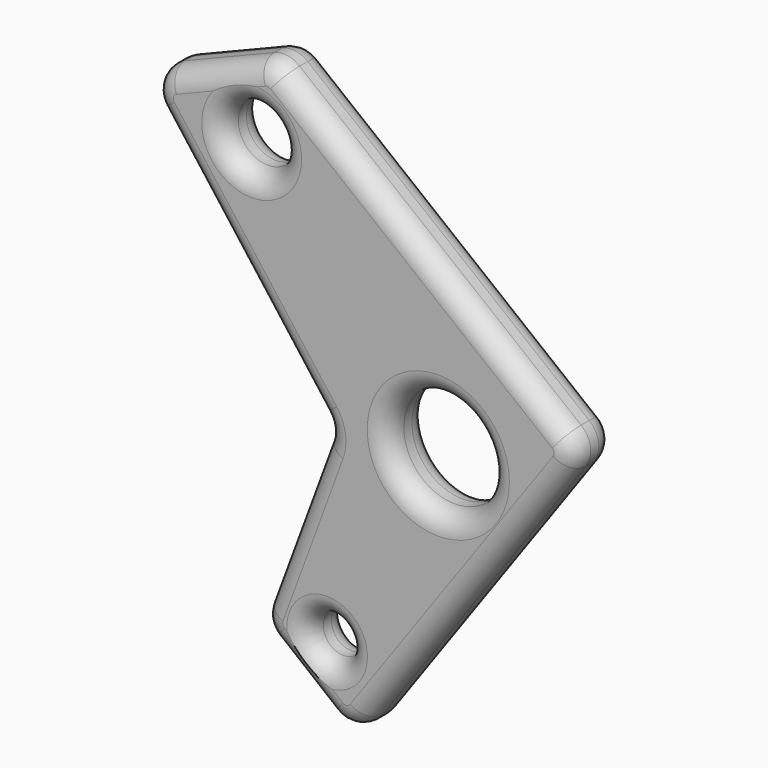
from build123d import *

# Parameters (mm, degrees)
F0_R         = 5.0114511668
F0_R_2       = 12.7
F0_R_3       = 7.4050061566
F1_DEPTH     = 12.7
F2_T1_DEPTH  = 67.4832294606
F2_T3_DEPTH  = 43.3480770651
F2_T5_DEPTH  = 18.6902227842
F2_T7_DEPTH  = 87.4726302362
F2_T9_DEPTH  = 90.1056698852
F2_T11_DEPTH = 24.0510688963
F2_T14_ANGLE = 104.9172533531
F2_T16_ANGLE = 57.3091059371
F2_T18_ANGLE = 71.4094727033
F2_T20_ANGLE = 93.3635037829
F2_T22_ANGLE = 86.9511700386
F2_T24_ANGLE = 60.6677060592
F3_T1_DEPTH  = 67.4832294606
F3_T3_DEPTH  = 43.3480770651
F3_T5_DEPTH  = 18.6902227842
F3_T7_DEPTH  = 87.4726302362
F3_T9_DEPTH  = 90.1056698852
F3_T11_DEPTH = 24.0510688963
F3_T14_ANGLE = 104.9172533531
F3_T16_ANGLE = 57.3091059371
F3_T18_ANGLE = 71.4094727033
F3_T20_ANGLE = 93.3635037829
F3_T22_ANGLE = 86.9511700386
F3_T24_ANGLE = 60.6677060592


# Not quite as in the source:
# - a fillet or chamfer that OpenCascade refuses, or shapes differently, is made with other operations: its cross-section is extruded or revolved along the edge and cut away or added


with BuildPart() as f1:
    # F0 (on Front) → F1 (new body)
    with BuildSketch(Plane.XZ):
        with BuildLine():
            Line((-70.0973556896, 53.2575167822), (-29.4707006051, -0.6262577244))
            ThreePointArc((-29.4707006051, -0.6262577244), (-28.258510501, -3.5258173929), (-28.5852000675, -6.6515373175))
            Line((-28.5852000675, -6.6515373175), (-43.6199162753, -47.3088010447))
            ThreePointArc((-43.6199162753, -47.3088010447), (-43.7857787204, -51.1986473183), (-41.6503181511, -54.4541384548))
            Line((-41.6503181511, -54.4541384548), (-27.101605684, -66.1869724377))
            ThreePointArc((-27.101605684, -66.1869724377), (-22.2538851697, -67.5353399701), (-17.947095407, -64.9334077788))
            Line((-17.947095407, -64.9334077788), (32.8746118318, 6.2607992451))
            ThreePointArc((32.8746118318, 6.2607992451), (33.9952305909, 10.8289222441), (31.6653512614, 14.9148978249))
            Line((31.6653512614, 14.9148978249), (-38.7836697055, 71.0928934304))
            ThreePointArc((-38.7836697055, 71.0928934304), (-41.8330514714, 72.4126619619), (-45.1314974688, 72.0116979572))
            Line((-45.1314974688, 72.0116979572), (-67.4158361597, 62.9639267308))
            ThreePointArc((-67.4158361597, 62.9639267308), (-71.1477537613, 58.7713096023), (-70.0973556896, 53.2575167822))
        make_face()
        with Locations((-27.8284879681, -50.1332112049)):
            Circle(F0_R, mode=Mode.SUBTRACT)
        Circle(F0_R_2, mode=Mode.SUBTRACT)
        with Locations((-46.6999868111, 54.0848947769)):
            Circle(F0_R_3, mode=Mode.SUBTRACT)
    extrude(amount=F1_DEPTH)

    # F2: fillet of radius 5.08 on 15 edges, made by hand

    # F2_s2 → F2_t1 (cut)
    with BuildSketch(Plane(origin=(-51.0068312032, 0, 67.6511660912), x_dir=(0, 1, 0), z_dir=(0.6020259464, 0, -0.7984765243))):
        with BuildLine():
            ThreePointArc((-7.62, -23.9086859864), (-11.2121024484, -22.4207884348), (-12.7, -18.8286859864))
            Line((-12.7, -18.8286859864), (-12.7, -23.9086859864))
            Line((-12.7, -23.9086859864), (-7.62, -23.9086859864))
        make_face()
    extrude(amount=F2_T1_DEPTH, mode=Mode.SUBTRACT)

    # F2_s4 → F2_t3 (cut)
    with BuildSketch(Plane(origin=(-5.6024752773, 0, -15.1503567959), x_dir=(0, 1, 0), z_dir=(-0.3468369816, 0, -0.9379254278))):
        with BuildLine():
            ThreePointArc((-7.62, -24.5037868769), (-11.2121024484, -23.0158893253), (-12.7, -19.4237868769))
            Line((-12.7, -19.4237868769), (-12.7, -24.5037868769))
            Line((-12.7, -24.5037868769), (-7.62, -24.5037868769))
        make_face()
    extrude(amount=F2_T3_DEPTH, mode=Mode.SUBTRACT)

    # F2_s6 → F2_t5 (cut)
    with BuildSketch(Plane(origin=(1.3720089605, 0, -1.1064589662), x_dir=(0, 1, 0), z_dir=(0.7784130042, 0, -0.6277524949))):
        with BuildLine():
            ThreePointArc((-7.62, -68.5339006399), (-11.2121024484, -67.0460030883), (-12.7, -63.4539006399))
            Line((-12.7, -63.4539006399), (-12.7, -68.5339006399))
            Line((-12.7, -68.5339006399), (-7.62, -68.5339006399))
        make_face()
    extrude(amount=F2_T5_DEPTH, mode=Mode.SUBTRACT)

    # F2_s8 → F2_t7 (cut)
    with BuildSketch(Plane(origin=(-36.7638756291, 0, -51.5011225467), x_dir=(0, 1, 0), z_dir=(0.5810012469, 0, 0.8139026668))):
        with BuildLine():
            ThreePointArc((-7.62, -23.1192020728), (-11.2121024484, -21.6313045212), (-12.7, -18.0392020728))
            Line((-12.7, -18.0392020728), (-12.7, -23.1192020728))
            Line((-12.7, -23.1192020728), (-7.62, -23.1192020728))
        make_face()
    extrude(amount=F2_T7_DEPTH, mode=Mode.SUBTRACT)

    # F2_s10 → F2_t9 (cut)
    with BuildSketch(Plane(origin=(12.0862587165, 0, -9.6379166061), x_dir=(0, 1, 0), z_dir=(-0.7818489231, 0, 0.6234679313))):
        with BuildLine():
            ThreePointArc((-7.62, -31.4035278491), (-11.2121024484, -29.9156302975), (-12.7, -26.3235278491))
            Line((-12.7, -26.3235278491), (-12.7, -31.4035278491))
            Line((-12.7, -31.4035278491), (-7.62, -31.4035278491))
        make_face()
    extrude(amount=F2_T9_DEPTH, mode=Mode.SUBTRACT)

    # F2_s12 → F2_t11 (cut)
    with BuildSketch(Plane(origin=(-13.6444260696, 0, -5.5398388665), x_dir=(0, 1, 0), z_dir=(-0.9265425494, 0, -0.3761899841))):
        with BuildLine():
            ThreePointArc((-7.62, -83.6999195282), (-11.2121024484, -82.2120219766), (-12.7, -78.6199195282))
            Line((-12.7, -78.6199195282), (-12.7, -83.6999195282))
            Line((-12.7, -83.6999195282), (-7.62, -83.6999195282))
        make_face()
    extrude(amount=F2_T11_DEPTH, mode=Mode.SUBTRACT)

    # F2_s13 → F2_t14 (revolve, cut)
    with BuildSketch(Plane(origin=(-35.9287647604, 0, -14.587610093), x_dir=(0, 1, 0), z_dir=(0.9265425494, 0, 0.3761899841))):
        with BuildLine():
            ThreePointArc((-7.62, 83.6999195282), (-11.2121024484, 82.2120219766), (-12.7, 78.6199195282))
            Line((-12.7, 78.6199195282), (-12.7, 83.6999195282))
            Line((-12.7, 83.6999195282), (-7.62, 83.6999195282))
        make_face()
    revolve(axis=Axis((-65.0270297604, -12.7, 57.0803815421), (0, -1, 0)), revolution_arc=F2_T14_ANGLE, mode=Mode.SUBTRACT)

    # F2_s15 → F2_t16 (revolve, cut)
    with BuildSketch(Plane(origin=(-10.3801761187, 0, 13.7673915846), x_dir=(0, 1, 0), z_dir=(-0.6020259464, 0, 0.7984765243))):
        with BuildLine():
            ThreePointArc((-7.62, 23.9086859864), (-11.2121024484, 22.4207884348), (-12.7, 18.8286859864))
            Line((-12.7, 18.8286859864), (-12.7, 23.9086859864))
            Line((-12.7, 23.9086859864), (-7.62, 23.9086859864))
        make_face()
    revolve(axis=Axis((-34.5410265343, -12.7, -4.4491224843), (0, 1, 0)), revolution_arc=F2_T16_ANGLE, mode=Mode.SUBTRACT)

    # F2_s17 → F2_t18 (revolve, cut)
    with BuildSketch(Plane(origin=(-20.6371914851, 0, -55.8076205231), x_dir=(0, 1, 0), z_dir=(0.3468369816, 0, 0.9379254278))):
        with BuildLine():
            ThreePointArc((-7.62, 24.5037868769), (-11.2121024484, 23.0158893253), (-12.7, 19.4237868769))
            Line((-12.7, 19.4237868769), (-12.7, 24.5037868769))
            Line((-12.7, 24.5037868769), (-7.62, 24.5037868769))
        make_face()
    revolve(axis=Axis((-37.6640898085, -12.7, -49.5112158779), (0, -1, 0)), revolution_arc=F2_T18_ANGLE, mode=Mode.SUBTRACT)

    # F2_s19 → F2_t20 (revolve, cut)
    with BuildSketch(Plane(origin=(15.9207214276, 0, -12.8392929492), x_dir=(0, 1, 0), z_dir=(-0.7784130042, 0, 0.6277524949))):
        with BuildLine():
            ThreePointArc((-7.62, 68.5339006399), (-11.2121024484, 67.0460030883), (-12.7, 63.4539006399))
            Line((-12.7, 63.4539006399), (-12.7, 68.5339006399))
            Line((-12.7, 68.5339006399), (-7.62, 68.5339006399))
        make_face()
    revolve(axis=Axis((-23.1153773414, -12.7, -61.2440498609), (0, -1, 0)), revolution_arc=F2_T20_ANGLE, mode=Mode.SUBTRACT)

    # F2_s21 → F2_t22 (revolve, cut)
    with BuildSketch(Plane(origin=(14.0578316098, 0, 19.6930844773), x_dir=(0, 1, 0), z_dir=(-0.5810012469, 0, -0.8139026668))):
        with BuildLine():
            ThreePointArc((-7.62, 23.1192020728), (-11.2121024484, 21.6313045212), (-12.7, 18.0392020728))
            Line((-12.7, 18.0392020728), (-12.7, 23.1192020728))
            Line((-12.7, 23.1192020728), (-7.62, 23.1192020728))
        make_face()
    revolve(axis=Axis((27.7063298974, -12.7, 9.9501571631), (0, -1, 0)), revolution_arc=F2_T22_ANGLE, mode=Mode.SUBTRACT)

    # F2_s23 → F2_t24 (revolve, cut)
    with BuildSketch(Plane(origin=(-58.3627622504, 0, 46.5400789994), x_dir=(0, 1, 0), z_dir=(0.7818489231, 0, -0.6234679313))):
        with BuildLine():
            ThreePointArc((-7.62, 31.4035278491), (-11.2121024484, 29.9156302975), (-12.7, 26.3235278491))
            Line((-12.7, 26.3235278491), (-12.7, 31.4035278491))
            Line((-12.7, 31.4035278491), (-7.62, 31.4035278491))
        make_face()
    revolve(axis=Axis((-42.7426910696, -12.7, 66.1281527686), (0, -1, 0)), revolution_arc=F2_T24_ANGLE, mode=Mode.SUBTRACT)

    # F2_s25 → F2_t26 (revolve, cut)
    with BuildSketch(Plane.XY.offset(-50.1332112049)):
        with BuildLine():
            ThreePointArc((-22.8170368014, -7.62), (-21.3291392498, -11.2121024484), (-17.7370368014, -12.7))
            Line((-17.7370368014, -12.7), (-22.8170368014, -12.7))
            Line((-22.8170368014, -12.7), (-22.8170368014, -7.62))
        make_face()
    revolve(axis=Axis((-27.8284879681, -12.7, -50.1332112049), (0, -1, 0)), mode=Mode.SUBTRACT)

    # F2_s27 → F2_t28 (revolve, cut)
    with BuildSketch(Plane.XY):
        with BuildLine():
            ThreePointArc((12.7, -7.62), (14.1878975516, -11.2121024484), (17.78, -12.7))
            Line((17.78, -12.7), (12.7, -12.7))
            Line((12.7, -12.7), (12.7, -7.62))
        make_face()
    revolve(axis=Axis((0, -12.7, 0), (0, -1, 0)), mode=Mode.SUBTRACT)

    # F2_s29 → F2_t30 (revolve, cut)
    with BuildSketch(Plane.XY.offset(54.0848947769)):
        with BuildLine():
            ThreePointArc((-39.2949806544, -7.62), (-37.8070831029, -11.2121024484), (-34.2149806544, -12.7))
            Line((-34.2149806544, -12.7), (-39.2949806544, -12.7))
            Line((-39.2949806544, -12.7), (-39.2949806544, -7.62))
        make_face()
    revolve(axis=Axis((-46.6999868111, -12.7, 54.0848947769), (0, -1, 0)), mode=Mode.SUBTRACT)

    # F3: fillet of radius 5.08 on 15 edges, made by hand

    # F3_s2 → F3_t1 (cut)
    with BuildSketch(Plane(origin=(-51.0068312032, 0, 67.6511660912), x_dir=(0, 1, 0), z_dir=(0.6020259464, 0, -0.7984765243))):
        with BuildLine():
            ThreePointArc((0, -18.8286859864), (-1.4878975516, -22.4207884348), (-5.08, -23.9086859864))
            Line((-5.08, -23.9086859864), (0, -23.9086859864))
            Line((0, -23.9086859864), (0, -18.8286859864))
        make_face()
    extrude(amount=F3_T1_DEPTH, mode=Mode.SUBTRACT)

    # F3_s4 → F3_t3 (cut)
    with BuildSketch(Plane(origin=(-5.6024752773, 0, -15.1503567959), x_dir=(0, 1, 0), z_dir=(-0.3468369816, 0, -0.9379254278))):
        with BuildLine():
            ThreePointArc((0, -19.4237868769), (-1.4878975516, -23.0158893253), (-5.08, -24.5037868769))
            Line((-5.08, -24.5037868769), (0, -24.5037868769))
            Line((0, -24.5037868769), (0, -19.4237868769))
        make_face()
    extrude(amount=F3_T3_DEPTH, mode=Mode.SUBTRACT)

    # F3_s6 → F3_t5 (cut)
    with BuildSketch(Plane(origin=(1.3720089605, 0, -1.1064589662), x_dir=(0, 1, 0), z_dir=(0.7784130042, 0, -0.6277524949))):
        with BuildLine():
            ThreePointArc((0, -63.4539006399), (-1.4878975516, -67.0460030883), (-5.08, -68.5339006399))
            Line((-5.08, -68.5339006399), (0, -68.5339006399))
            Line((0, -68.5339006399), (0, -63.4539006399))
        make_face()
    extrude(amount=F3_T5_DEPTH, mode=Mode.SUBTRACT)

    # F3_s8 → F3_t7 (cut)
    with BuildSketch(Plane(origin=(-36.7638756291, 0, -51.5011225467), x_dir=(0, 1, 0), z_dir=(0.5810012469, 0, 0.8139026668))):
        with BuildLine():
            ThreePointArc((0, -18.0392020728), (-1.4878975516, -21.6313045212), (-5.08, -23.1192020728))
            Line((-5.08, -23.1192020728), (0, -23.1192020728))
            Line((0, -23.1192020728), (0, -18.0392020728))
        make_face()
    extrude(amount=F3_T7_DEPTH, mode=Mode.SUBTRACT)

    # F3_s10 → F3_t9 (cut)
    with BuildSketch(Plane(origin=(12.0862587165, 0, -9.6379166061), x_dir=(0, 1, 0), z_dir=(-0.7818489231, 0, 0.6234679313))):
        with BuildLine():
            ThreePointArc((0, -26.3235278491), (-1.4878975516, -29.9156302975), (-5.08, -31.4035278491))
            Line((-5.08, -31.4035278491), (0, -31.4035278491))
            Line((0, -31.4035278491), (0, -26.3235278491))
        make_face()
    extrude(amount=F3_T9_DEPTH, mode=Mode.SUBTRACT)

    # F3_s12 → F3_t11 (cut)
    with BuildSketch(Plane(origin=(-13.6444260696, 0, -5.5398388665), x_dir=(0, 1, 0), z_dir=(-0.9265425494, 0, -0.3761899841))):
        with BuildLine():
            ThreePointArc((0, -78.6199195282), (-1.4878975516, -82.2120219766), (-5.08, -83.6999195282))
            Line((-5.08, -83.6999195282), (0, -83.6999195282))
            Line((0, -83.6999195282), (0, -78.6199195282))
        make_face()
    extrude(amount=F3_T11_DEPTH, mode=Mode.SUBTRACT)

    # F3_s13 → F3_t14 (revolve, cut)
    with BuildSketch(Plane(origin=(-35.9287647604, 0, -14.587610093), x_dir=(0, 1, 0), z_dir=(0.9265425494, 0, 0.3761899841))):
        with BuildLine():
            ThreePointArc((-5.08, 83.6999195282), (-1.4878975516, 82.2120219766), (0, 78.6199195282))
            Line((0, 78.6199195282), (0, 83.6999195282))
            Line((0, 83.6999195282), (-5.08, 83.6999195282))
        make_face()
    revolve(axis=Axis((-65.0270297604, 0, 57.0803815421), (0, -1, 0)), revolution_arc=F3_T14_ANGLE, mode=Mode.SUBTRACT)

    # F3_s15 → F3_t16 (revolve, cut)
    with BuildSketch(Plane(origin=(-10.3801761187, 0, 13.7673915846), x_dir=(0, 1, 0), z_dir=(-0.6020259464, 0, 0.7984765243))):
        with BuildLine():
            ThreePointArc((0, 18.8286859864), (-1.4878975516, 22.4207884348), (-5.08, 23.9086859864))
            Line((-5.08, 23.9086859864), (0, 23.9086859864))
            Line((0, 23.9086859864), (0, 18.8286859864))
        make_face()
    revolve(axis=Axis((-34.5410265343, 0, -4.4491224843), (0, 1, 0)), revolution_arc=F3_T16_ANGLE, mode=Mode.SUBTRACT)

    # F3_s17 → F3_t18 (revolve, cut)
    with BuildSketch(Plane(origin=(-20.6371914851, 0, -55.8076205231), x_dir=(0, 1, 0), z_dir=(0.3468369816, 0, 0.9379254278))):
        with BuildLine():
            ThreePointArc((0, 19.4237868769), (-1.4878975516, 23.0158893253), (-5.08, 24.5037868769))
            Line((-5.08, 24.5037868769), (0, 24.5037868769))
            Line((0, 24.5037868769), (0, 19.4237868769))
        make_face()
    revolve(axis=Axis((-37.6640898085, 0, -49.5112158779), (0, -1, 0)), revolution_arc=F3_T18_ANGLE, mode=Mode.SUBTRACT)

    # F3_s19 → F3_t20 (revolve, cut)
    with BuildSketch(Plane(origin=(15.9207214276, 0, -12.8392929492), x_dir=(0, 1, 0), z_dir=(-0.7784130042, 0, 0.6277524949))):
        with BuildLine():
            ThreePointArc((0, 63.4539006399), (-1.4878975516, 67.0460030883), (-5.08, 68.5339006399))
            Line((-5.08, 68.5339006399), (0, 68.5339006399))
            Line((0, 68.5339006399), (0, 63.4539006399))
        make_face()
    revolve(axis=Axis((-23.1153773414, 0, -61.2440498609), (0, -1, 0)), revolution_arc=F3_T20_ANGLE, mode=Mode.SUBTRACT)

    # F3_s21 → F3_t22 (revolve, cut)
    with BuildSketch(Plane(origin=(14.0578316098, 0, 19.6930844773), x_dir=(0, 1, 0), z_dir=(-0.5810012469, 0, -0.8139026668))):
        with BuildLine():
            ThreePointArc((0, 18.0392020728), (-1.4878975516, 21.6313045212), (-5.08, 23.1192020728))
            Line((-5.08, 23.1192020728), (0, 23.1192020728))
            Line((0, 23.1192020728), (0, 18.0392020728))
        make_face()
    revolve(axis=Axis((27.7063298974, 0, 9.9501571631), (0, -1, 0)), revolution_arc=F3_T22_ANGLE, mode=Mode.SUBTRACT)

    # F3_s23 → F3_t24 (revolve, cut)
    with BuildSketch(Plane(origin=(-58.3627622504, 0, 46.5400789994), x_dir=(0, 1, 0), z_dir=(0.7818489231, 0, -0.6234679313))):
        with BuildLine():
            ThreePointArc((0, 26.3235278491), (-1.4878975516, 29.9156302975), (-5.08, 31.4035278491))
            Line((-5.08, 31.4035278491), (0, 31.4035278491))
            Line((0, 31.4035278491), (0, 26.3235278491))
        make_face()
    revolve(axis=Axis((-42.7426910696, 0, 66.1281527686), (0, -1, 0)), revolution_arc=F3_T24_ANGLE, mode=Mode.SUBTRACT)

    # F3_s25 → F3_t26 (revolve, cut)
    with BuildSketch(Plane.XY.offset(-50.1332112049)):
        with BuildLine():
            ThreePointArc((-17.7370368014, 0), (-21.3291392498, -1.4878975516), (-22.8170368014, -5.08))
            Line((-22.8170368014, -5.08), (-22.8170368014, 0))
            Line((-22.8170368014, 0), (-17.7370368014, 0))
        make_face()
    revolve(axis=Axis((-27.8284879681, 0, -50.1332112049), (0, -1, 0)), mode=Mode.SUBTRACT)

    # F3_s27 → F3_t28 (revolve, cut)
    with BuildSketch(Plane.XY):
        with BuildLine():
            ThreePointArc((17.78, 0), (14.1878975516, -1.4878975516), (12.7, -5.08))
            Line((12.7, -5.08), (12.7, 0))
            Line((12.7, 0), (17.78, 0))
        make_face()
    revolve(axis=Axis((0, 0, 0), (0, -1, 0)), mode=Mode.SUBTRACT)

    # F3_s29 → F3_t30 (revolve, cut)
    with BuildSketch(Plane.XY.offset(54.0848947769)):
        with BuildLine():
            ThreePointArc((-34.2149806544, 0), (-37.8070831029, -1.4878975516), (-39.2949806544, -5.08))
            Line((-39.2949806544, -5.08), (-39.2949806544, 0))
            Line((-39.2949806544, 0), (-34.2149806544, 0))
        make_face()
    revolve(axis=Axis((-46.6999868111, 0, 54.0848947769), (0, -1, 0)), mode=Mode.SUBTRACT)


solid = f1.part
